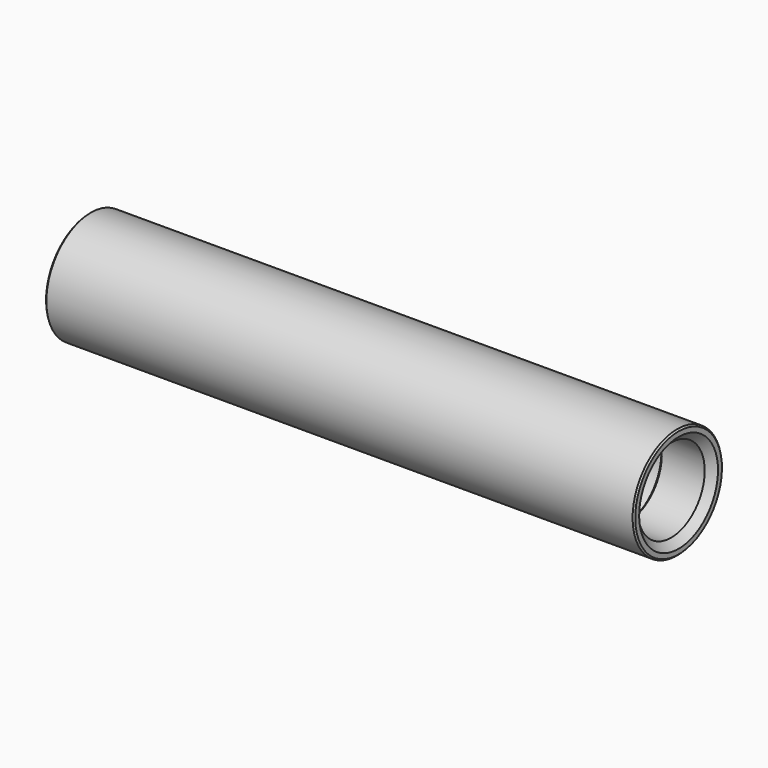
from build123d import *

# Parameters (mm, degrees)
F2_SIZE  = 0.5
F3_SIZE  = 2.5
F4_SIZE  = 2.5
F5_SIZE2 = 1.09999
F5_SIZE  = 0.99999
F6_SIZE2 = 1.06
F6_SIZE  = 1


# Not quite as in the source:
# - a fillet or chamfer is up to 0.001 mm smaller than in the source, because OpenCascade refuses the exact size


with BuildPart() as f1:
    # F0 (on Front) → F1 (revolve)
    with BuildSketch(Plane.XZ):
        Polygon((0, 18.8), (0, 14.15), (17, 14.15), (17, 15.25), (23, 15.25), (23, 12.5), (99.5, 12.5), (99.5, 18.8), align=None)
        Polygon((199, 18.8), (99.5, 18.8), (99.5, 12.5), (176, 12.5), (176, 15.25), (182, 15.25), (182, 14.15), (199, 14.15), align=None)
    revolve(axis=Axis((99.5, 0, 0), (-1, 0, 0)))

    # F2
    f2_edges = [f1.edges().sort_by_distance(p)[0] for p in [
        (199, 0, -18.8),
        (0, 0, -18.8),
    ]]
    chamfer(f2_edges, length=F2_SIZE)

    # F3
    f3_edges = [f1.edges().sort_by_distance(p)[0] for p in [
        (0, 0, -14.15),
    ]]
    chamfer(f3_edges, length=F3_SIZE)

    # F4
    f4_edges = [f1.edges().sort_by_distance(p)[0] for p in [
        (199, 0, -14.15),
    ]]
    chamfer(f4_edges, length=F4_SIZE)

    # F5 (size 1 and 1.1 in the source; OpenCascade refuses exactly that, so slightly less here)
    f5_edges = [f1.edges().sort_by_distance(p)[0] for p in [
        (17, 0, -14.15),
    ]]
    chamfer(f5_edges, length=F5_SIZE, length2=F5_SIZE2)

    # F6
    f6_edges = [f1.edges().sort_by_distance(p)[0] for p in [
        (182, 0, -15.25),
    ]]
    chamfer(f6_edges, length=F6_SIZE, length2=F6_SIZE2)


solid = f1.part
